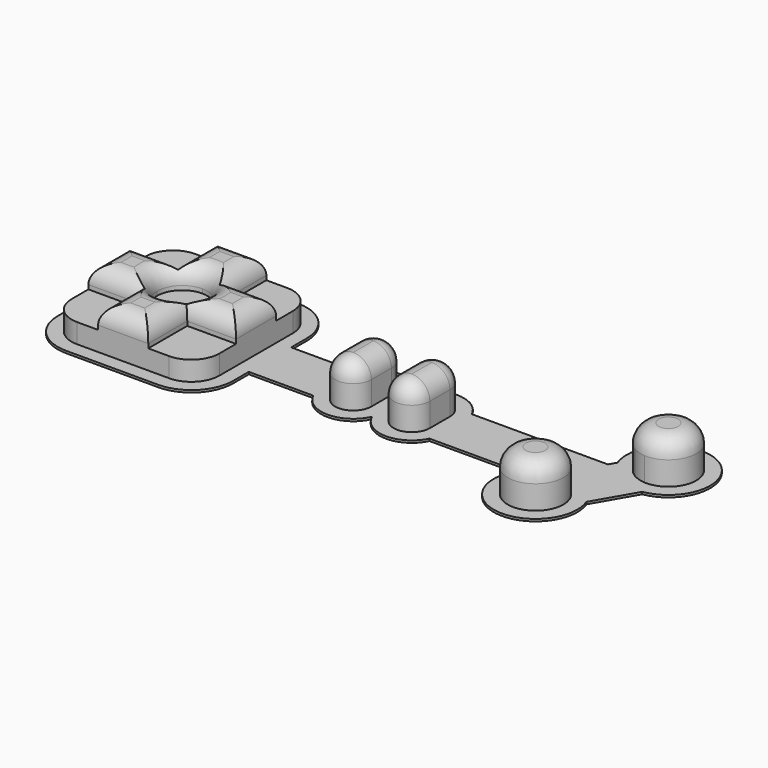
from build123d import *

# Parameters (mm, degrees)
F0_W         = 16
F0_H         = 4.5
F0_W_2       = 6.5
F0_W_3       = 4
F1_DEPTH     = 0.4
F2_W         = 6.5
F2_H         = 2.25
F3_DEPTH     = 7.5
F5_DEPTH     = 4
F6_T1_DEPTH  = 16.875
F6_T3_DEPTH  = 16.875
F6_T5_DEPTH  = 25.25
F6_T7_DEPTH  = 16.875
F6_T9_DEPTH  = 25.25
F6_T11_DEPTH = 16.875
F6_T13_DEPTH = 4.5
F6_T18_ANGLE = 180
F6_T20_ANGLE = 180
F6_T26_ANGLE = 180
F6_T28_ANGLE = 180
F6_T33_DEPTH = 25
F6_T37_DEPTH = 25
F6_T44_DEPTH = 25
F6_T48_DEPTH = 25
F6_T55_DEPTH = 25
F6_T59_DEPTH = 25
F6_T66_DEPTH = 25
F6_T70_DEPTH = 25


# Not quite as in the source:
# - a fillet or chamfer that OpenCascade refuses, or shapes differently, is made with other operations: its cross-section is extruded or revolved along the edge and cut away or added
# - the program builds the solid bodies; features that only make, move or delete a surface that nothing else refers to are left out


with BuildPart() as f1:
    # F0 (on Top) → F1 (new body)
    with BuildSketch(Plane.XY):
        with BuildLine():
            ThreePointArc((37.8219210467, -4.7500002533), (41.5209457211, -7.8065188161), (46.25, -6.9934167973))
            ThreePointArc((46.25, -6.9934167973), (47.3607749493, -5.9978186662), (48.1780789533, -4.7500002533))
            Line((48.1780789533, -4.7500002533), (63.9480825285, -4.7500002533))
            ThreePointArc((63.9480825285, -4.7500002533), (69.6474452613, -16.1274569996), (77.3637438503, -6.0087617448))
            Line((77.3637438503, -6.0087617448), (81.5596503471, 1.2587614915))
            ThreePointArc((81.5596503471, 1.2587614915), (84.098076338, 15.1554447856), (73.3324085724, 6.0087617448))
            Line((73.3324085724, 6.0087617448), (72.6056622864, 4.7500002533))
            Line((72.6056622864, 4.7500002533), (48.1780789533, 4.7500002533))
            ThreePointArc((48.1780789533, 4.7500002533), (43, 8.0000002533), (37.8219210467, 4.7500002533))
            Line((37.8219210467, 4.7500002533), (37.6780789533, 4.7500002533))
            ThreePointArc((37.6780789533, 4.7500002533), (32.5, 8.0000002533), (27.3219210467, 4.7500002533))
            Line((27.3219210467, 4.7500002533), (15.7500002533, 4.7500002533))
            Line((15.7500002533, 4.7500002533), (15.7500002533, 8.25))
            ThreePointArc((15.7500002533, 8.25), (13.553301038, 13.553301038), (8.25, 15.7500002533))
            Line((8.25, 15.7500002533), (-8.25, 15.7500002533))
            ThreePointArc((-8.25, 15.7500002533), (-13.553301038, 13.553301038), (-15.7500002533, 8.25))
            Line((-15.7500002533, 8.25), (-15.7500002533, -8.25))
            ThreePointArc((-15.7500002533, -8.25), (-13.553301038, -13.553301038), (-8.25, -15.7500002533))
            Line((-8.25, -15.7500002533), (8.25, -15.7500002533))
            ThreePointArc((8.25, -15.7500002533), (13.553301038, -13.553301038), (15.7500002533, -8.25))
            Line((15.7500002533, -8.25), (15.7500002533, -4.7500002533))
            Line((15.7500002533, -4.7500002533), (27.3219210467, -4.7500002533))
            ThreePointArc((27.3219210467, -4.7500002533), (32.5, -8.0000002533), (37.6780789533, -4.7500002533))
            Line((37.6780789533, -4.7500002533), (37.8219210467, -4.7500002533))
        make_face()
        with BuildLine():
            ThreePointArc((13.25, -8.25), (11.7855339059, -11.7855339059), (8.25, -13.25))
            Line((8.25, -13.25), (4.5, -13.25))
            Line((4.5, -13.25), (-4.5, -13.25))
            Line((-4.5, -13.25), (-8.25, -13.25))
            ThreePointArc((-8.25, -13.25), (-11.7855339059, -11.7855339059), (-13.25, -8.25))
            Line((-13.25, -8.25), (-13.25, -4.5))
            Line((-13.25, -4.5), (-13.25, 4.5))
            Line((-13.25, 4.5), (-13.25, 8.25))
            ThreePointArc((-13.25, 8.25), (-11.7855339059, 11.7855339059), (-8.25, 13.25))
            Line((-8.25, 13.25), (-4.5, 13.25))
            Line((-4.5, 13.25), (4.5, 13.25))
            Line((4.5, 13.25), (8.25, 13.25))
            ThreePointArc((8.25, 13.25), (11.7855339059, 11.7855339059), (13.25, 8.25))
            Line((13.25, 8.25), (13.25, 4.5))
            Line((13.25, 4.5), (13.25, 2.25))
            Line((13.25, 2.25), (29.25, 2.25))
            ThreePointArc((29.25, 2.25), (32.5, 5.5), (35.75, 2.25))
            Line((35.75, 2.25), (39.75, 2.25))
            ThreePointArc((39.75, 2.25), (43, 5.5), (46.25, 2.25))
            Line((46.25, 2.25), (74.0490381057, 2.25))
            Line((74.0490381057, 2.25), (76.1669476654, 5.9183269633))
            ThreePointArc((76.1669476654, 5.9183269633), (82.8480762114, 12.9903810568), (80.0640619824, 3.6683269633))
            Line((80.0640619824, 3.6683269633), (74.5292047573, -5.9183269633))
            ThreePointArc((74.5292047573, -5.9183269633), (67.8480762114, -12.9903810568), (70.6320904403, -3.6683269633))
            Line((70.6320904403, -3.6683269633), (71.4509618943, -2.25))
            Line((71.4509618943, -2.25), (46.25, -2.25))
            ThreePointArc((46.25, -2.25), (43, -5.5), (39.75, -2.25))
            Line((39.75, -2.25), (35.75, -2.25))
            ThreePointArc((35.75, -2.25), (32.5, -5.5), (29.25, -2.25))
            Line((29.25, -2.25), (13.25, -2.25))
            Line((13.25, -2.25), (13.25, -4.5))
            Line((13.25, -4.5), (13.25, -8.25))
        make_face(mode=Mode.SUBTRACT)
        Polygon((46.25, 2.25), (46.25, -2.25), (71.4509618943, -2.25), (74.0490381057, 2.25), align=None)
        Polygon((-4.5, -13.25), (4.5, -13.25), (4.5, -4.5), (0, -4.5), (-4.5, -4.5), align=None)
        Polygon((4.5, 0), (4.5, -4.5), (13.25, -4.5), (13.25, -2.25), (13.25, 2.25), (13.25, 4.5), (4.5, 4.5), align=None)
        Polygon((-4.5, 4.5), (0, 4.5), (4.5, 4.5), (4.5, 13.25), (-4.5, 13.25), align=None)
        Polygon((-13.25, -4.5), (-4.5, -4.5), (-4.5, 0), (-4.5, 4.5), (-13.25, 4.5), align=None)
        with BuildLine():
            ThreePointArc((80.0640619824, 3.6683269633), (82.8480762114, 12.9903810568), (76.1669476654, 5.9183269633))
            ThreePointArc((76.1669476654, 5.9183269633), (77.8480762114, 4.3301270189), (80.0640619824, 3.6683269633))
        make_face()
        with BuildLine():
            ThreePointArc((74.5292047573, -5.9183269633), (72.8480762114, -4.3301270189), (70.6320904403, -3.6683269633))
            ThreePointArc((70.6320904403, -3.6683269633), (67.8480762114, -12.9903810568), (74.5292047573, -5.9183269633))
        make_face()
        with Locations((21.25, 0)):
            Rectangle(F0_W, F0_H)
        with BuildLine():
            Line((-8.25, -13.25), (-4.5, -13.25))
            Line((-4.5, -13.25), (-4.5, -4.5))
            Line((-4.5, -4.5), (-13.25, -4.5))
            Line((-13.25, -4.5), (-13.25, -8.25))
            ThreePointArc((-13.25, -8.25), (-11.7855339059, -11.7855339059), (-8.25, -13.25))
        make_face()
        with BuildLine():
            Line((4.5, 13.25), (4.5, 4.5))
            Line((4.5, 4.5), (13.25, 4.5))
            Line((13.25, 4.5), (13.25, 8.25))
            ThreePointArc((13.25, 8.25), (11.7855339059, 11.7855339059), (8.25, 13.25))
            Line((8.25, 13.25), (4.5, 13.25))
        make_face()
        with BuildLine():
            Line((4.5, -13.25), (8.25, -13.25))
            ThreePointArc((8.25, -13.25), (11.7855339059, -11.7855339059), (13.25, -8.25))
            Line((13.25, -8.25), (13.25, -4.5))
            Line((13.25, -4.5), (4.5, -4.5))
            Line((4.5, -4.5), (4.5, -13.25))
        make_face()
        with BuildLine():
            Line((-13.25, 4.5), (-4.5, 4.5))
            Line((-4.5, 4.5), (-4.5, 13.25))
            Line((-4.5, 13.25), (-8.25, 13.25))
            ThreePointArc((-8.25, 13.25), (-11.7855339059, 11.7855339059), (-13.25, 8.25))
            Line((-13.25, 8.25), (-13.25, 4.5))
        make_face()
        with BuildLine():
            ThreePointArc((0, -4.5), (3.1819805153, -3.1819805153), (4.5, 0))
            ThreePointArc((4.5, 0), (3.1819805153, 3.1819805153), (0, 4.5))
            ThreePointArc((0, 4.5), (-3.1819805153, 3.1819805153), (-4.5, 0))
            ThreePointArc((-4.5, 0), (-3.1819805153, -3.1819805153), (0, -4.5))
        make_face()
        with BuildLine():
            Line((74.0490381057, 2.25), (71.4509618943, -2.25))
            Line((71.4509618943, -2.25), (70.6320904403, -3.6683269633))
            ThreePointArc((70.6320904403, -3.6683269633), (72.8480762114, -4.3301270189), (74.5292047573, -5.9183269633))
            Line((74.5292047573, -5.9183269633), (80.0640619824, 3.6683269633))
            ThreePointArc((80.0640619824, 3.6683269633), (77.8480762114, 4.3301270189), (76.1669476654, 5.9183269633))
            Line((76.1669476654, 5.9183269633), (74.0490381057, 2.25))
        make_face()
        with Locations((32.5, 0)):
            Rectangle(F0_W_2, F0_H)
        with Locations((43, 0)):
            Rectangle(F0_W_2, F0_H)
        with Locations((37.75, 0)):
            Rectangle(F0_W_3, F0_H)
        with BuildLine():
            Line((35.75, -2.25), (29.25, -2.25))
            ThreePointArc((29.25, -2.25), (32.5, -5.5), (35.75, -2.25))
        make_face()
        with BuildLine():
            Line((46.25, -2.25), (39.75, -2.25))
            ThreePointArc((39.75, -2.25), (43, -5.5), (46.25, -2.25))
        make_face()
        with BuildLine():
            ThreePointArc((46.25, 2.25), (43, 5.5), (39.75, 2.25))
            Line((39.75, 2.25), (46.25, 2.25))
        make_face()
        with BuildLine():
            ThreePointArc((35.75, 2.25), (32.5, 5.5), (29.25, 2.25))
            Line((29.25, 2.25), (35.75, 2.25))
        make_face()
        with BuildLine():
            ThreePointArc((0, 4.5), (3.1819805153, 3.1819805153), (4.5, 0))
            Line((4.5, 0), (4.5, 4.5))
            Line((4.5, 4.5), (0, 4.5))
        make_face()
        with BuildLine():
            Line((0, -4.5), (4.5, -4.5))
            Line((4.5, -4.5), (4.5, 0))
            ThreePointArc((4.5, 0), (3.1819805153, -3.1819805153), (0, -4.5))
        make_face()
        with BuildLine():
            Line((-4.5, 4.5), (-4.5, 0))
            ThreePointArc((-4.5, 0), (-3.1819805153, 3.1819805153), (0, 4.5))
            Line((0, 4.5), (-4.5, 4.5))
        make_face()
        with BuildLine():
            Line((-4.5, 0), (-4.5, -4.5))
            Line((-4.5, -4.5), (0, -4.5))
            ThreePointArc((0, -4.5), (-3.1819805153, -3.1819805153), (-4.5, 0))
        make_face()
    extrude(amount=F1_DEPTH)

    # F2 (on face) → F3 (join)
    with BuildSketch(Plane.XY.offset(0.4)):
        with BuildLine():
            Line((-13.25, 4.5), (-4.5, 4.5))
            Line((-4.5, 4.5), (-4.5, 13.25))
            Line((-4.5, 13.25), (-8.25, 13.25))
            ThreePointArc((-8.25, 13.25), (-11.7855339059, 11.7855339059), (-13.25, 8.25))
            Line((-13.25, 8.25), (-13.25, 4.5))
        make_face()
        Polygon((-4.5, 4.5), (0, 4.5), (4.5, 4.5), (4.5, 13.25), (-4.5, 13.25), align=None)
        with BuildLine():
            Line((4.5, 13.25), (4.5, 4.5))
            Line((4.5, 4.5), (13.25, 4.5))
            Line((13.25, 4.5), (13.25, 8.25))
            ThreePointArc((13.25, 8.25), (11.7855339059, 11.7855339059), (8.25, 13.25))
            Line((8.25, 13.25), (4.5, 13.25))
        make_face()
        Polygon((4.5, 0), (4.5, -4.5), (13.25, -4.5), (13.25, -2.25), (13.25, 2.25), (13.25, 4.5), (4.5, 4.5), align=None)
        with BuildLine():
            Line((4.5, -13.25), (8.25, -13.25))
            ThreePointArc((8.25, -13.25), (11.7855339059, -11.7855339059), (13.25, -8.25))
            Line((13.25, -8.25), (13.25, -4.5))
            Line((13.25, -4.5), (4.5, -4.5))
            Line((4.5, -4.5), (4.5, -13.25))
        make_face()
        Polygon((-4.5, -13.25), (4.5, -13.25), (4.5, -4.5), (0, -4.5), (-4.5, -4.5), align=None)
        with BuildLine():
            Line((-8.25, -13.25), (-4.5, -13.25))
            Line((-4.5, -13.25), (-4.5, -4.5))
            Line((-4.5, -4.5), (-13.25, -4.5))
            Line((-13.25, -4.5), (-13.25, -8.25))
            ThreePointArc((-13.25, -8.25), (-11.7855339059, -11.7855339059), (-8.25, -13.25))
        make_face()
        with BuildLine():
            Line((-4.5, 0), (-4.5, -4.5))
            Line((-4.5, -4.5), (0, -4.5))
            ThreePointArc((0, -4.5), (-3.1819805153, -3.1819805153), (-4.5, 0))
        make_face()
        with BuildLine():
            Line((0, -4.5), (4.5, -4.5))
            Line((4.5, -4.5), (4.5, 0))
            ThreePointArc((4.5, 0), (3.1819805153, -3.1819805153), (0, -4.5))
        make_face()
        with BuildLine():
            Line((-4.5, 4.5), (-4.5, 0))
            ThreePointArc((-4.5, 0), (-3.1819805153, 3.1819805153), (0, 4.5))
            Line((0, 4.5), (-4.5, 4.5))
        make_face()
        Polygon((-13.25, -4.5), (-4.5, -4.5), (-4.5, 0), (-4.5, 4.5), (-13.25, 4.5), align=None)
        with BuildLine():
            ThreePointArc((0, 4.5), (3.1819805153, 3.1819805153), (4.5, 0))
            Line((4.5, 0), (4.5, 4.5))
            Line((4.5, 4.5), (0, 4.5))
        make_face()
        with BuildLine():
            ThreePointArc((0, -4.5), (3.1819805153, -3.1819805153), (4.5, 0))
            ThreePointArc((4.5, 0), (3.1819805153, 3.1819805153), (0, 4.5))
            ThreePointArc((0, 4.5), (-3.1819805153, 3.1819805153), (-4.5, 0))
            ThreePointArc((-4.5, 0), (-3.1819805153, -3.1819805153), (0, -4.5))
        make_face()
        with Locations((32.5, -1.125)):
            Rectangle(F2_W, F2_H)
        with Locations((32.5, 1.125)):
            Rectangle(F2_W, F2_H)
        with BuildLine():
            ThreePointArc((35.75, 2.25), (32.5, 5.5), (29.25, 2.25))
            Line((29.25, 2.25), (35.75, 2.25))
        make_face()
        with BuildLine():
            Line((35.75, -2.25), (29.25, -2.25))
            ThreePointArc((29.25, -2.25), (32.5, -5.5), (35.75, -2.25))
        make_face()
        with BuildLine():
            Line((46.25, -2.25), (39.75, -2.25))
            ThreePointArc((39.75, -2.25), (43, -5.5), (46.25, -2.25))
        make_face()
        with Locations((43, -1.125)):
            Rectangle(F2_W, F2_H)
        with Locations((43, 1.125)):
            Rectangle(F2_W, F2_H)
        with BuildLine():
            ThreePointArc((46.25, 2.25), (43, 5.5), (39.75, 2.25))
            Line((39.75, 2.25), (46.25, 2.25))
        make_face()
        with BuildLine():
            ThreePointArc((72.8480762114, -4.3301270189), (71.7788727151, -3.8693437522), (70.6320904403, -3.6683269633))
            ThreePointArc((70.6320904403, -3.6683269633), (67.8480762114, -12.9903810568), (74.5292047573, -5.9183269633))
            ThreePointArc((74.5292047573, -5.9183269633), (73.7817279741, -5.0256927751), (72.8480762114, -4.3301270189))
        make_face()
        with BuildLine():
            ThreePointArc((80.0640619824, 3.6683269633), (82.8480762114, 12.9903810568), (76.1669476654, 5.9183269633))
            ThreePointArc((76.1669476654, 5.9183269633), (76.9144244486, 5.0256927751), (77.8480762114, 4.3301270189))
            ThreePointArc((77.8480762114, 4.3301270189), (78.9172797076, 3.8693437522), (80.0640619824, 3.6683269633))
        make_face()
    extrude(amount=F3_DEPTH)

    # F4 (on face) → F5 (cut)
    with BuildSketch(Plane.XY.offset(7.9)):
        with BuildLine():
            Line((4.5, 13.25), (4.5, 4.5))
            Line((4.5, 4.5), (13.25, 4.5))
            Line((13.25, 4.5), (13.25, 8.25))
            ThreePointArc((13.25, 8.25), (11.7855339059, 11.7855339059), (8.25, 13.25))
            Line((8.25, 13.25), (4.5, 13.25))
        make_face()
        with BuildLine():
            Line((-13.25, 4.5), (-4.5, 4.5))
            Line((-4.5, 4.5), (-4.5, 13.25))
            Line((-4.5, 13.25), (-8.25, 13.25))
            ThreePointArc((-8.25, 13.25), (-11.7855339059, 11.7855339059), (-13.25, 8.25))
            Line((-13.25, 8.25), (-13.25, 4.5))
        make_face()
        with BuildLine():
            Line((-8.25, -13.25), (-4.5, -13.25))
            Line((-4.5, -13.25), (-4.5, -4.5))
            Line((-4.5, -4.5), (-13.25, -4.5))
            Line((-13.25, -4.5), (-13.25, -8.25))
            ThreePointArc((-13.25, -8.25), (-11.7855339059, -11.7855339059), (-8.25, -13.25))
        make_face()
        with BuildLine():
            Line((4.5, -13.25), (8.25, -13.25))
            ThreePointArc((8.25, -13.25), (11.7855339059, -11.7855339059), (13.25, -8.25))
            Line((13.25, -8.25), (13.25, -4.5))
            Line((13.25, -4.5), (4.5, -4.5))
            Line((4.5, -4.5), (4.5, -13.25))
        make_face()
        with BuildLine():
            ThreePointArc((0, -4.5), (3.1819805153, -3.1819805153), (4.5, 0))
            ThreePointArc((4.5, 0), (3.1819805153, 3.1819805153), (0, 4.5))
            ThreePointArc((0, 4.5), (-3.1819805153, 3.1819805153), (-4.5, 0))
            ThreePointArc((-4.5, 0), (-3.1819805153, -3.1819805153), (0, -4.5))
        make_face()
    extrude(amount=-F5_DEPTH, mode=Mode.SUBTRACT)

    # F6: fillet of radius 3.25 on 23 edges, made by hand

    # F6_s2 → F6_t1 (cut)
    with BuildSketch(Plane.YZ.offset(-21.375)):
        with BuildLine():
            ThreePointArc((1.25, 7.9), (3.5480970389, 6.9480970389), (4.5, 4.65))
            Line((4.5, 4.65), (4.5, 7.9))
            Line((4.5, 7.9), (1.25, 7.9))
        make_face()
        with BuildLine():
            ThreePointArc((-4.5, 4.65), (-3.5480970389, 6.9480970389), (-1.25, 7.9))
            Line((-1.25, 7.9), (-4.5, 7.9))
            Line((-4.5, 7.9), (-4.5, 4.65))
        make_face()
    extrude(amount=F6_T1_DEPTH, mode=Mode.SUBTRACT)

    # F6_s4 → F6_t3 (cut)
    with BuildSketch(Plane.XZ.offset(-21.375)):
        with BuildLine():
            ThreePointArc((-1.25, 7.9), (-3.5480970389, 6.9480970389), (-4.5, 4.65))
            Line((-4.5, 4.65), (-4.5, 7.9))
            Line((-4.5, 7.9), (-1.25, 7.9))
        make_face()
        with BuildLine():
            ThreePointArc((1.25, 7.9), (3.5480970389, 6.9480970389), (4.5, 4.65))
            Line((4.5, 4.65), (4.5, 7.9))
            Line((4.5, 7.9), (1.25, 7.9))
        make_face()
    extrude(amount=F6_T3_DEPTH, mode=Mode.SUBTRACT)

    # F6_s6 → F6_t5 (cut)
    with BuildSketch(Plane.YZ.offset(-12.625)):
        with BuildLine():
            ThreePointArc((13.25, 4.65), (12.2980970389, 6.9480970389), (10, 7.9))
            Line((10, 7.9), (13.25, 7.9))
            Line((13.25, 7.9), (13.25, 4.65))
        make_face()
        with BuildLine():
            ThreePointArc((-13.25, 4.65), (-12.2980970389, 6.9480970389), (-10, 7.9))
            Line((-10, 7.9), (-13.25, 7.9))
            Line((-13.25, 7.9), (-13.25, 4.65))
        make_face()
    extrude(amount=F6_T5_DEPTH, mode=Mode.SUBTRACT)

    # F6_s8 → F6_t7 (cut)
    with BuildSketch(Plane.YZ.offset(4.5)):
        with BuildLine():
            ThreePointArc((1.25, 7.9), (3.5480970389, 6.9480970389), (4.5, 4.65))
            Line((4.5, 4.65), (4.5, 7.9))
            Line((4.5, 7.9), (1.25, 7.9))
        make_face()
        with BuildLine():
            ThreePointArc((-1.25, 7.9), (-3.5480970389, 6.9480970389), (-4.5, 4.65))
            Line((-4.5, 4.65), (-4.5, 7.9))
            Line((-4.5, 7.9), (-1.25, 7.9))
        make_face()
    extrude(amount=F6_T7_DEPTH, mode=Mode.SUBTRACT)

    # F6_s10 → F6_t9 (cut)
    with BuildSketch(Plane.XZ.offset(-12.625)):
        with BuildLine():
            ThreePointArc((13.25, 4.65), (12.2980970389, 6.9480970389), (10, 7.9))
            Line((10, 7.9), (13.25, 7.9))
            Line((13.25, 7.9), (13.25, 4.65))
        make_face()
        with BuildLine():
            ThreePointArc((-13.25, 4.65), (-12.2980970389, 6.9480970389), (-10, 7.9))
            Line((-10, 7.9), (-13.25, 7.9))
            Line((-13.25, 7.9), (-13.25, 4.65))
        make_face()
    extrude(amount=F6_T9_DEPTH, mode=Mode.SUBTRACT)

    # F6_s12 → F6_t11 (cut)
    with BuildSketch(Plane.XZ.offset(4.5)):
        with BuildLine():
            ThreePointArc((1.25, 7.9), (3.5480970389, 6.9480970389), (4.5, 4.65))
            Line((4.5, 4.65), (4.5, 7.9))
            Line((4.5, 7.9), (1.25, 7.9))
        make_face()
        with BuildLine():
            ThreePointArc((-1.25, 7.9), (-3.5480970389, 6.9480970389), (-4.5, 4.65))
            Line((-4.5, 4.65), (-4.5, 7.9))
            Line((-4.5, 7.9), (-1.25, 7.9))
        make_face()
    extrude(amount=F6_T11_DEPTH, mode=Mode.SUBTRACT)

    # F6_s14 → F6_t13 (cut)
    with BuildSketch(Plane.XZ.offset(-2.25)):
        with BuildLine():
            ThreePointArc((35.75, 4.65), (34.7980970389, 6.9480970389), (32.5, 7.9))
            Line((32.5, 7.9), (35.75, 7.9))
            Line((35.75, 7.9), (35.75, 4.65))
        make_face()
        with BuildLine():
            ThreePointArc((46.25, 4.65), (45.2980970389, 6.9480970389), (43, 7.9))
            Line((43, 7.9), (46.25, 7.9))
            Line((46.25, 7.9), (46.25, 4.65))
        make_face()
        with BuildLine():
            ThreePointArc((39.75, 4.65), (40.7019029611, 6.9480970389), (43, 7.9))
            Line((43, 7.9), (39.75, 7.9))
            Line((39.75, 7.9), (39.75, 4.65))
        make_face()
        with BuildLine():
            ThreePointArc((29.25, 4.65), (30.2019029611, 6.9480970389), (32.5, 7.9))
            Line((32.5, 7.9), (29.25, 7.9))
            Line((29.25, 7.9), (29.25, 4.65))
        make_face()
    extrude(amount=F6_T13_DEPTH, mode=Mode.SUBTRACT)

    # F6_s15 → F6_t16 (revolve, cut)
    with BuildSketch(Plane.XZ):
        with BuildLine():
            ThreePointArc((7.75, 7.9), (5.4519029611, 6.9480970389), (4.5, 4.65))
            Line((4.5, 4.65), (4.5, 7.9))
            Line((4.5, 7.9), (7.75, 7.9))
        make_face()
    revolve(axis=Axis((0, 0, 7.9), (0, 0, 1)), mode=Mode.SUBTRACT)

    # F6_s17 → F6_t18 (revolve, cut)
    with BuildSketch(Plane.XZ.offset(2.25)):
        with BuildLine():
            ThreePointArc((39.75, 4.65), (40.7019029611, 6.9480970389), (43, 7.9))
            Line((43, 7.9), (39.75, 7.9))
            Line((39.75, 7.9), (39.75, 4.65))
        make_face()
    revolve(axis=Axis((43, -2.25, 7.9), (0, 0, 1)), revolution_arc=F6_T18_ANGLE, mode=Mode.SUBTRACT)

    # F6_s19 → F6_t20 (revolve, cut)
    with BuildSketch(Plane.XZ.offset(-2.25)):
        with BuildLine():
            ThreePointArc((46.25, 4.65), (45.2980970389, 6.9480970389), (43, 7.9))
            Line((43, 7.9), (46.25, 7.9))
            Line((46.25, 7.9), (46.25, 4.65))
        make_face()
    revolve(axis=Axis((43, 2.25, 7.9), (0, 0, 1)), revolution_arc=F6_T20_ANGLE, mode=Mode.SUBTRACT)

    # F6_s21 → F6_t22 (revolve, cut)
    with BuildSketch(Plane(origin=(56.5110571585, -32.6266740627, 0), x_dir=(0, 0, 1), z_dir=(0.8660254038, -0.5, 0))):
        with BuildLine():
            ThreePointArc((4.65, -32.6740381057), (6.9480970389, -31.7221351445), (7.9, -29.4240381057))
            Line((7.9, -29.4240381057), (7.9, -32.6740381057))
            Line((7.9, -32.6740381057), (4.65, -32.6740381057))
        make_face()
    revolve(axis=Axis((70.3480762114, -8.6602540378, 7.9), (0, 0, 1)), mode=Mode.SUBTRACT)

    # F6_s23 → F6_t24 (revolve, cut)
    with BuildSketch(Plane(origin=(20.1914336424, -30.7896516902, 0), x_dir=(0, 0, 1), z_dir=(-0.5483854149, 0.8362257092, 0))):
        with BuildLine():
            ThreePointArc((4.65, 66.9382840157), (6.9480970389, 67.8901869769), (7.9, 70.1882840157))
            Line((7.9, 70.1882840157), (7.9, 66.9382840157))
            Line((7.9, 66.9382840157), (4.65, 66.9382840157))
        make_face()
    revolve(axis=Axis((80.3480762114, 8.6602540378, 7.9), (0, 0, 1)), mode=Mode.SUBTRACT)

    # F6_s25 → F6_t26 (revolve, cut)
    with BuildSketch(Plane.XZ.offset(-2.25)):
        with BuildLine():
            ThreePointArc((35.75, 4.65), (34.7980970389, 6.9480970389), (32.5, 7.9))
            Line((32.5, 7.9), (35.75, 7.9))
            Line((35.75, 7.9), (35.75, 4.65))
        make_face()
    revolve(axis=Axis((32.5, 2.25, 7.9), (0, 0, 1)), revolution_arc=F6_T26_ANGLE, mode=Mode.SUBTRACT)

    # F6_s27 → F6_t28 (revolve, cut)
    with BuildSketch(Plane.XZ.offset(2.25)):
        with BuildLine():
            ThreePointArc((29.25, 4.65), (30.2019029611, 6.9480970389), (32.5, 7.9))
            Line((32.5, 7.9), (29.25, 7.9))
            Line((29.25, 7.9), (29.25, 4.65))
        make_face()
    revolve(axis=Axis((32.5, -2.25, 7.9), (0, 0, 1)), revolution_arc=F6_T28_ANGLE, mode=Mode.SUBTRACT)


with BuildPart() as f6_tool31:
    # F6_s32 → F6_t33 (new body)
    with BuildSketch(Plane.YZ.offset(-21.375)):
        with BuildLine():
            ThreePointArc((1.25, 7.9), (3.5480970389, 6.9480970389), (4.5, 4.65))
            Line((4.5, 4.65), (4.5, 7.9))
            Line((4.5, 7.9), (1.25, 7.9))
        make_face()
    extrude(amount=F6_T33_DEPTH)

    split(bisect_by=Plane.YZ.offset(-4.5), keep=Keep.TOP)


with BuildPart() as f6_tool35:
    # F6_s36 → F6_t37 (new body)
    with BuildSketch(Plane.XZ.offset(3.625)):
        with BuildLine():
            ThreePointArc((-1.25, 7.9), (-3.5480970389, 6.9480970389), (-4.5, 4.65))
            Line((-4.5, 4.65), (-4.5, 7.9))
            Line((-4.5, 7.9), (-1.25, 7.9))
        make_face()
    extrude(amount=-F6_T37_DEPTH)

    split(bisect_by=Plane.XZ.offset(-4.5), keep=Keep.TOP)


with BuildPart() as f6_tool31_1:
    add(f6_tool31.part)

    # F6_t39: intersect F6_tool35
    add(f6_tool35.part, mode=Mode.INTERSECT)


with BuildPart() as f1_1:
    add(f1.part)

    # F6_t29: cut F6_tool31
    add(f6_tool31_1.part, mode=Mode.SUBTRACT)


with BuildPart() as f6_tool42:
    # F6_s43 → F6_t44 (new body)
    with BuildSketch(Plane.XZ.offset(-21.375)):
        with BuildLine():
            ThreePointArc((1.25, 7.9), (3.5480970389, 6.9480970389), (4.5, 4.65))
            Line((4.5, 4.65), (4.5, 7.9))
            Line((4.5, 7.9), (1.25, 7.9))
        make_face()
    extrude(amount=F6_T44_DEPTH)

    split(bisect_by=Plane.XZ.offset(-4.5), keep=Keep.TOP)


with BuildPart() as f6_tool46:
    # F6_s47 → F6_t48 (new body)
    with BuildSketch(Plane.YZ.offset(-3.625)):
        with BuildLine():
            ThreePointArc((1.25, 7.9), (3.5480970389, 6.9480970389), (4.5, 4.65))
            Line((4.5, 4.65), (4.5, 7.9))
            Line((4.5, 7.9), (1.25, 7.9))
        make_face()
    extrude(amount=F6_T48_DEPTH)

    split(bisect_by=Plane.YZ.offset(4.5), keep=Keep.BOTTOM)


with BuildPart() as f6_tool42_1:
    add(f6_tool42.part)

    # F6_t50: intersect F6_tool46
    add(f6_tool46.part, mode=Mode.INTERSECT)


with BuildPart() as f1_2:
    add(f1_1.part)

    # F6_t40: cut F6_tool42
    add(f6_tool42_1.part, mode=Mode.SUBTRACT)


with BuildPart() as f6_tool53:
    # F6_s54 → F6_t55 (new body)
    with BuildSketch(Plane.YZ.offset(21.375)):
        with BuildLine():
            ThreePointArc((-1.25, 7.9), (-3.5480970389, 6.9480970389), (-4.5, 4.65))
            Line((-4.5, 4.65), (-4.5, 7.9))
            Line((-4.5, 7.9), (-1.25, 7.9))
        make_face()
    extrude(amount=-F6_T55_DEPTH)

    split(bisect_by=Plane.YZ.offset(4.5), keep=Keep.BOTTOM)


with BuildPart() as f6_tool57:
    # F6_s58 → F6_t59 (new body)
    with BuildSketch(Plane.XZ.offset(-3.625)):
        with BuildLine():
            ThreePointArc((1.25, 7.9), (3.5480970389, 6.9480970389), (4.5, 4.65))
            Line((4.5, 4.65), (4.5, 7.9))
            Line((4.5, 7.9), (1.25, 7.9))
        make_face()
    extrude(amount=F6_T59_DEPTH)

    split(bisect_by=Plane.XZ.offset(4.5), keep=Keep.BOTTOM)


with BuildPart() as f6_tool53_1:
    add(f6_tool53.part)

    # F6_t61: intersect F6_tool57
    add(f6_tool57.part, mode=Mode.INTERSECT)


with BuildPart() as f1_3:
    add(f1_2.part)

    # F6_t51: cut F6_tool53
    add(f6_tool53_1.part, mode=Mode.SUBTRACT)


with BuildPart() as f6_tool64:
    # F6_s65 → F6_t66 (new body)
    with BuildSketch(Plane.YZ.offset(3.625)):
        with BuildLine():
            ThreePointArc((-4.5, 4.65), (-3.5480970389, 6.9480970389), (-1.25, 7.9))
            Line((-1.25, 7.9), (-4.5, 7.9))
            Line((-4.5, 7.9), (-4.5, 4.65))
        make_face()
    extrude(amount=-F6_T66_DEPTH)

    split(bisect_by=Plane.YZ.offset(-4.5), keep=Keep.TOP)


with BuildPart() as f6_tool68:
    # F6_s69 → F6_t70 (new body)
    with BuildSketch(Plane.XZ.offset(21.375)):
        with BuildLine():
            ThreePointArc((-1.25, 7.9), (-3.5480970389, 6.9480970389), (-4.5, 4.65))
            Line((-4.5, 4.65), (-4.5, 7.9))
            Line((-4.5, 7.9), (-1.25, 7.9))
        make_face()
    extrude(amount=-F6_T70_DEPTH)

    split(bisect_by=Plane.XZ.offset(4.5), keep=Keep.BOTTOM)


with BuildPart() as f6_tool64_1:
    add(f6_tool64.part)

    # F6_t72: intersect F6_tool68
    add(f6_tool68.part, mode=Mode.INTERSECT)


with BuildPart() as f1_4:
    add(f1_3.part)

    # F6_t62: cut F6_tool64
    add(f6_tool64_1.part, mode=Mode.SUBTRACT)


solid = f1_4.part
